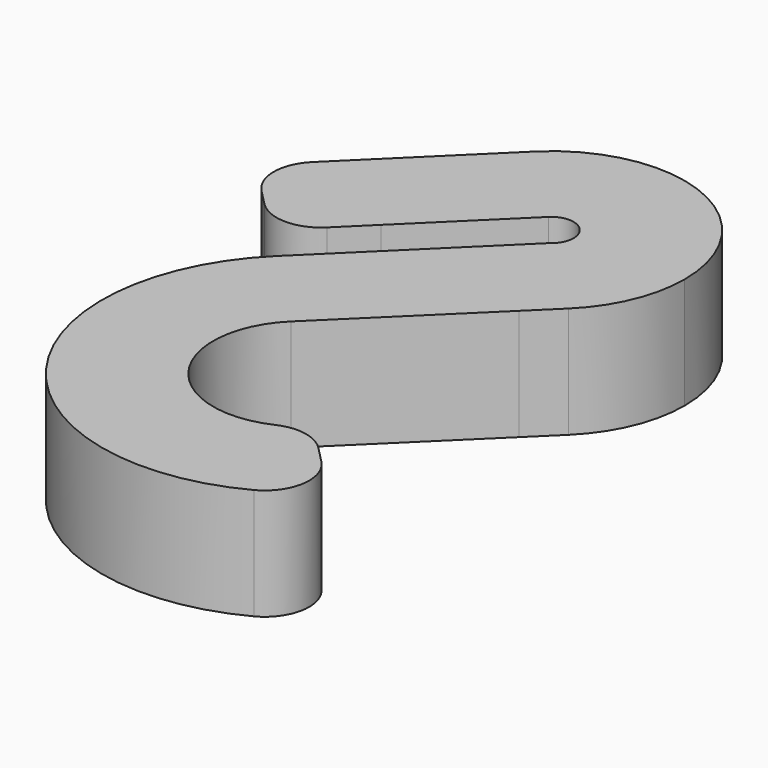
from build123d import *

# Parameters (mm, degrees)
F1_DEPTH = 5
F3_R     = 2


# Not quite as in the source:
# - a feature of the source that left no trace in its solid (it failed there, or was rolled back) is left out
# - a feature names something its author has since deleted; it is built from what else it names


with BuildPart() as f1:
    # F0 (on Top) → F1 (new body)
    with BuildSketch(Plane.XY):
        with BuildLine():
            ThreePointArc((1, 4.2856675661), (0.9540832917, 3.9861261291), (0.820549855, 3.7140926057))
            ThreePointArc((0.820549855, 3.7140926057), (0.7011095464, 3.5726139889), (0.5576336696, 3.4555804077))
            Line((0.5576336696, 3.4555804077), (-3.5314378692, -0.5649969839))
            ThreePointArc((-3.5314378692, -0.5649969839), (-3.0925503087, -0.8559404108), (-2.6298440658, -1.1072834062))
            ThreePointArc((-2.6298440658, -1.1072834062), (0, -0.714485053), (2.6298440658, -1.1072834062))
            ThreePointArc((2.6298440658, -1.1072834062), (3.4591021242, -0.6168432696), (4.1991729558, 0))
            ThreePointArc((4.1991729558, 0), (5.531502406, 1.961343765), (6, 4.2856675661))
            ThreePointArc((6, 4.2856675661), (2.4042381835, 9.7829067602), (-4.073212919, 8.6912250242))
            Line((-4.073212919, 8.6912250242), (-4.3361291045, 8.4327128262))
            ThreePointArc((-4.3361291045, 8.4327128262), (-5.9823120662, 4.7460395278), (-4.9195913989, 0.8509011303))
            Line((-4.9195913989, 0.8509011303), (-0.7011096797, 4.9987210123))
            ThreePointArc((-0.7011096797, 4.9987210123), (0.3865813759, 5.2079228669), (1, 4.2856675661))
        make_face()
        with BuildLine():
            ThreePointArc((-2.6298440658, -1.1072834062), (-3.0925503087, -0.8559404108), (-3.5314378692, -0.5649969839))
            Line((-3.5314378692, -0.5649969839), (-6.3099859173, -3.297002858))
            ThreePointArc((-6.3099859173, -3.297002858), (-4.6020493099, -1.9800722021), (-2.6298440658, -1.1072834062))
        make_face()
        with BuildLine():
            Line((-7.7001872259, -1.8831182213), (-4.9195913989, 0.8509011303))
            ThreePointArc((-4.9195913989, 0.8509011303), (-5.9823120662, 4.7460395278), (-4.3361291045, 8.4327128262))
            Line((-4.3361291045, 8.4327128262), (-11.2037486913, 1.6801295606))
            Line((-11.2037486913, 1.6801295606), (-7.7001872259, -1.8831182213))
        make_face()
        with BuildLine():
            ThreePointArc((2.6298440658, -1.1072834062), (0, -0.714485053), (-2.6298440658, -1.1072834062))
            ThreePointArc((-2.6298440658, -1.1072834062), (0, -1.7143324339), (2.6298440658, -1.1072834062))
        make_face()
        with BuildLine():
            ThreePointArc((2.6298440658, -1.1072834062), (0, -1.7143324339), (-2.6298440658, -1.1072834062))
            ThreePointArc((-2.6298440658, -1.1072834062), (-4.6020493099, -1.9800722021), (-6.3099859173, -3.297002858))
            ThreePointArc((-6.3099859173, -3.297002858), (-6.4229942249, -16.018860136), (6.2987594337, -16.1429864022))
            Line((6.2987594337, -16.1429864022), (2.7994486372, -12.5715967638))
            ThreePointArc((2.7994486372, -12.5715967638), (-2.8571117107, -12.5139336903), (-2.7994486372, -6.8573733423))
            Line((-2.7994486372, -6.8573733423), (2.9592441197, -1.2149042257))
            ThreePointArc((2.9592441197, -1.2149042257), (2.7950621185, -1.1595082703), (2.6298440658, -1.1072834062))
        make_face()
        with BuildLine():
            ThreePointArc((4.1991729558, 0), (3.4591021242, -0.6168432696), (2.6298440658, -1.1072834062))
            ThreePointArc((2.6298440658, -1.1072834062), (2.7950621185, -1.1595082703), (2.9592441197, -1.2149042257))
            Line((2.9592441197, -1.2149042257), (4.1991729558, 0))
        make_face()
    extrude(amount=F1_DEPTH)

    # F3
    f3_edges = [f1.edges().sort_by_distance(p)[0] for p in [
        (-11.203749, 1.68013, 2.5),
        (-7.700187, -1.883118, 2.5),
        (6.298759, -16.142986, 2.5),
        (2.799449, -12.571597, 2.5),
    ]]
    fillet(f3_edges, radius=F3_R)


solid = f1.part
